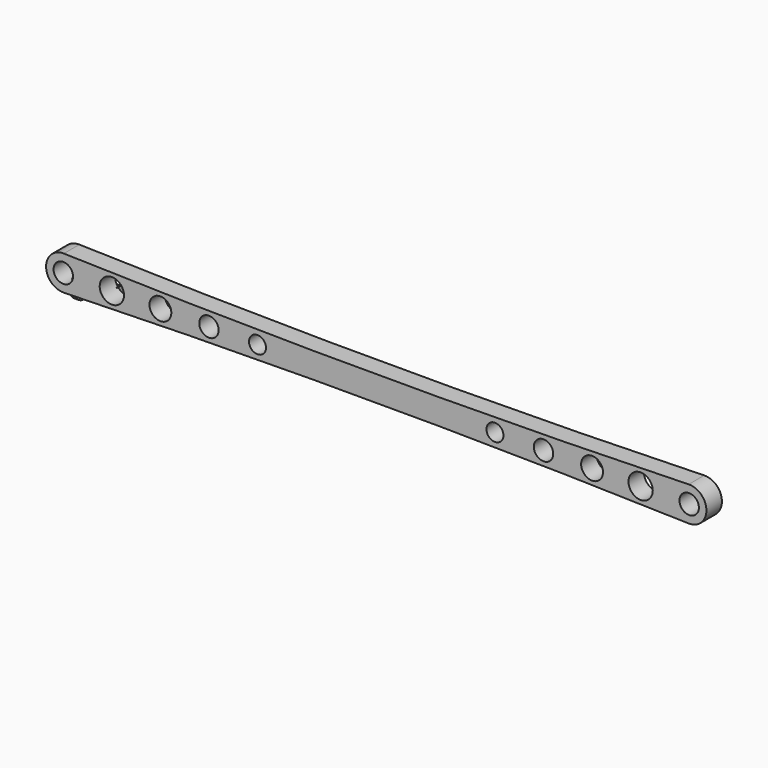
from build123d import *

# Parameters (mm, degrees)
F0_R     = 1
F0_R_2   = 1.25
F0_R_3   = 1.125
F0_R_4   = 0.875
F1_DEPTH = 2
F5_DEPTH = 0.75


with BuildPart() as f1:
    # F0 (on Front) → F1 (new body)
    with BuildSketch(Plane.XZ):
        with BuildLine():
            ThreePointArc((64.3489094749, 3.5436613707), (32.1744547374, 3.0632452956), (0, 3.5436613707))
            ThreePointArc((0, 3.5436613707), (-1.8255452626, 1.7718306853), (0, 0))
            ThreePointArc((0, 0), (32.1744547374, 0.4804160751), (64.3489094749, 0))
            ThreePointArc((64.3489094749, 0), (66.1744547374, 1.7718306853), (64.3489094749, 3.5436613707))
        make_face()
        with Locations((-0.0529243323, 1.7718306853)):
            Circle(F0_R, mode=Mode.SUBTRACT)
        with Locations((4.9470756677, 1.7718306853)):
            Circle(F0_R_2, mode=Mode.SUBTRACT)
        with Locations((9.9470756677, 1.7718306853)):
            Circle(F0_R_3, mode=Mode.SUBTRACT)
        with Locations((14.9470756677, 1.7718306853)):
            Circle(F0_R, mode=Mode.SUBTRACT)
        with Locations((19.9470756677, 1.7718306853)):
            Circle(F0_R_4, mode=Mode.SUBTRACT)
        with Locations((44.4018338072, 1.7718306853)):
            Circle(F0_R_4, mode=Mode.SUBTRACT)
        with Locations((49.4018338072, 1.7718306853)):
            Circle(F0_R, mode=Mode.SUBTRACT)
        with Locations((54.4018338072, 1.7718306853)):
            Circle(F0_R_3, mode=Mode.SUBTRACT)
        with Locations((59.4018338072, 1.7718306853)):
            Circle(F0_R_2, mode=Mode.SUBTRACT)
        with Locations((64.4018338072, 1.7718306853)):
            Circle(F0_R, mode=Mode.SUBTRACT)
    extrude(amount=F1_DEPTH)


with BuildPart() as f3:
    # F2 (on Front) → F3 (revolve)
    with BuildSketch(Plane.XZ):
        Polygon((0, 1.25), (0, 0), (4, 0), (4, 1), (0.5, 1), (0.5, 1.25), align=None)
    revolve(axis=Axis((1.7442880877, 0, 0), (1, 0, 0)))

    # F4 (on face) → F5 (cut)
    with BuildSketch(Plane(origin=(0, 0, 0), x_dir=(0, -1, 0), z_dir=(-1, 0, 0))):
        Polygon((0.3614844576, -0.7498537696), (0.8116411571, -0.1849062488), (0.6506155109, 0.5192794487), (-0.0003368852, 0.83243713), (-0.6510355999, 0.5187526738), (-0.8114912291, -0.1855631264), (-0.3608774115, -0.7501461076), align=None)
    extrude(amount=-F5_DEPTH, mode=Mode.SUBTRACT)


solid = Compound([f1.part, f3.part])
